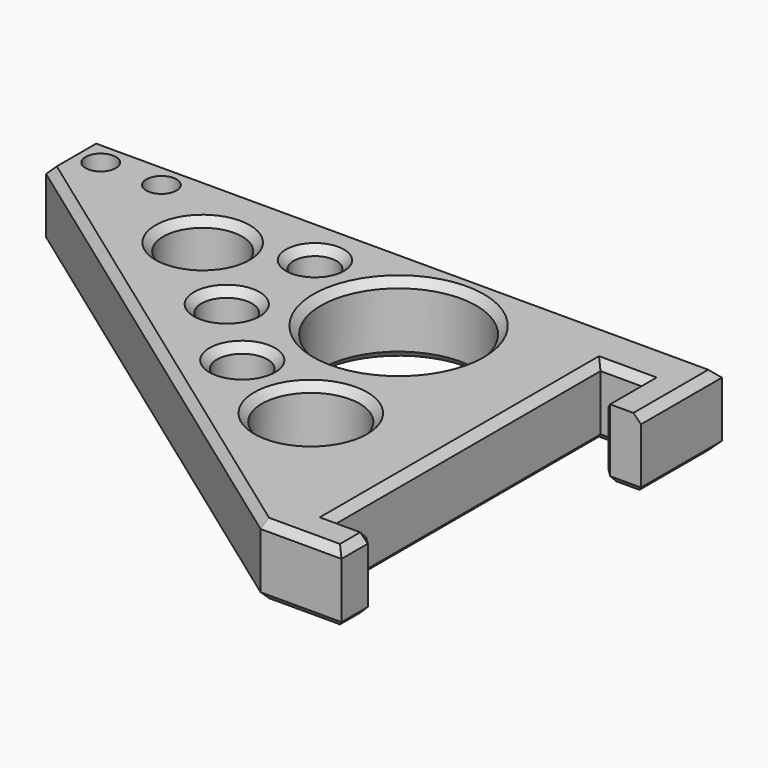
from build123d import *

# Parameters (mm, degrees)
F0_W     = 3.8
F0_H     = 5
F0_W_2   = 4
F0_H_2   = 4
F0_R     = 2.5006647493
F0_R_2   = 4.8327220748
F0_R_3   = 3.906097333
F0_R_4   = 2.1231290944
F0_R_5   = 7.6831288046
F0_W_3   = 12
F0_H_3   = 6
F0_R_6   = 1.5
F1_DEPTH = 7
F2_SIZE  = 0.75


# Not quite as in the source:
# - a feature names something its author has since deleted; it is built from what else it names


with BuildPart() as f1:
    # F0 (on Top) → F1 (new body)
    with BuildSketch(Plane.XY):
        Polygon((0, 10.6260057762), (0, 15.6260057762), (-4, 15.6260057762), (-4, -26.3739942238), (0, -26.3739942238), (0, -22.3739942238), align=None)
        Polygon((8, 15.6260057762), (0, 15.6260057762), (0, 10.6260057762), (4.2, 10.6260057762), (8, 10.6260057762), align=None)
        with Locations((6.1, 8.1260057762)):
            Rectangle(F0_W, F0_H)
        with Locations((2, -24.3739942238)):
            Rectangle(F0_W_2, F0_H_2)
        Polygon((-4, -26.3739942238), (-4, 15.6260057762), (-42, 15.6260057762), (-42, 9.6260057762), (-54, 9.6260057762), align=None)
        with Locations((-21.8336265534, -6.3459714875)):
            Circle(F0_R, mode=Mode.SUBTRACT)
        with Locations((-12.1693955734, -9.9561735988)):
            Circle(F0_R_2, mode=Mode.SUBTRACT)
        with Locations((-28.6096986383, 0.2079327387)):
            Circle(F0_R, mode=Mode.SUBTRACT)
        with Locations((-36.4965982735, 7.095086854)):
            Circle(F0_R_3, mode=Mode.SUBTRACT)
        with Locations((-27.8876554221, 10.2054132149)):
            Circle(F0_R_4, mode=Mode.SUBTRACT)
        with Locations((-16.008509323, 5.6881718338)):
            Circle(F0_R_5, mode=Mode.SUBTRACT)
        with Locations((-48, 12.6260057762)):
            Rectangle(F0_W_3, F0_H_3)
        with Locations((-51, 12.6260057762)):
            Circle(F0_R_6, mode=Mode.SUBTRACT)
        with Locations((-45, 12.6260057762)):
            Circle(F0_R_6, mode=Mode.SUBTRACT)
    extrude(amount=F1_DEPTH)

    # F2
    f2_edges = [f1.edges().sort_by_distance(p)[0] for p in [
        (4.2, 5.626006, 3.5),
        (4, -22.373994, 3.5),
        (-17.002118, -9.956174, 0),
        (-31.110363, 0.207933, 0),
        (-40.402696, 7.095087, 7),
        (-40.402696, 7.095087, 0),
        (-30.010785, 10.205413, 0),
        (-23.691638, 5.688172, 0),
        (0, -5.873994, 0),
        (2.1, 10.626006, 0),
        (4.2, 8.126006, 0),
        (6.1, 5.626006, 0),
        (8, 10.626006, 0),
        (-23, 15.626006, 0),
        (-54, 12.626006, 0),
        (-29, -8.373994, 0),
        (0, -26.373994, 0),
        (4, -24.373994, 0),
        (2, -22.373994, 0),
        (-23, 15.626006, 7),
        (-54, 12.626006, 7),
        (-29, -8.373994, 7),
        (-30.010785, 10.205413, 7),
        (-31.110363, 0.207933, 7),
        (-23.691638, 5.688172, 7),
        (-17.002118, -9.956174, 7),
        (0, -26.373994, 7),
        (4, -24.373994, 7),
        (2, -22.373994, 7),
        (0, -5.873994, 7),
        (8, 10.626006, 7),
        (2.1, 10.626006, 7),
        (4.2, 8.126006, 7),
        (-24.334291, -6.345971, 7),
        (-24.334291, -6.345971, 0),
    ]]
    chamfer(f2_edges, length=F2_SIZE)


solid = f1.part
